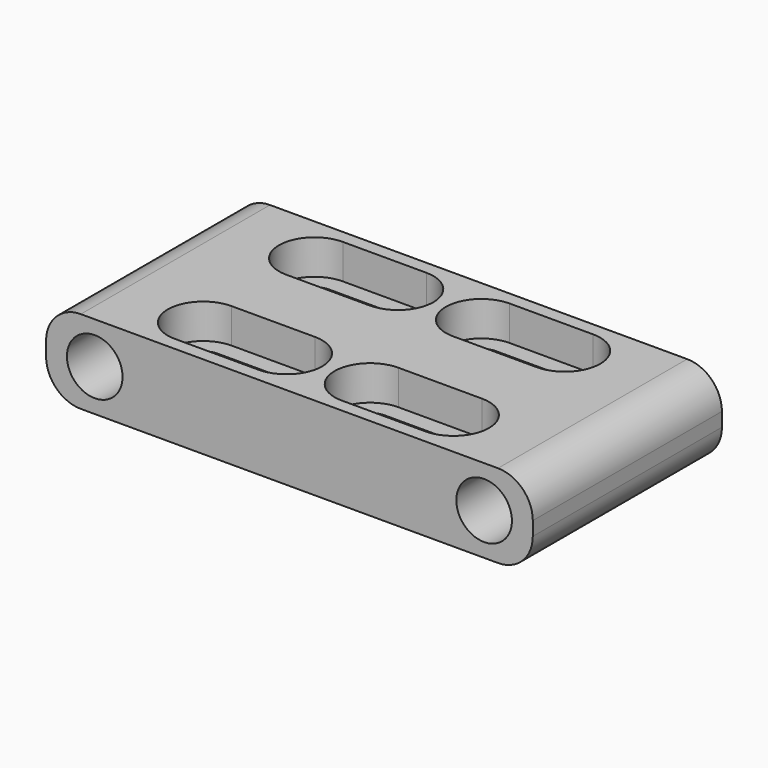
from build123d import *

# Parameters (mm, degrees)
F0_W     = 70
F0_H     = 34
F1_DEPTH = 12
F2_DEPTH = 7
F3_R     = 4
F4_DEPTH = 34.001
F5_R     = 5


# Not quite as in the source:
# - a feature names something its author has since deleted; it is built from what else it names


with BuildPart() as f1:
    # F0 (on Top) → F1 (new body)
    with BuildSketch(Plane.XY):
        Rectangle(F0_W, F0_H)
        with BuildLine():
            Line((-6, -15.1), (-18, -15.1))
            ThreePointArc((-18, -15.1), (-23.1, -10), (-18, -4.9))
            Line((-18, -4.9), (-6, -4.9))
            ThreePointArc((-6, -4.9), (-0.9, -10), (-6, -15.1))
        make_face(mode=Mode.SUBTRACT)
        with BuildLine():
            ThreePointArc((6, -15.1), (0.9, -10), (6, -4.9))
            Line((6, -4.9), (18, -4.9))
            ThreePointArc((18, -4.9), (23.1, -10), (18, -15.1))
            Line((18, -15.1), (6, -15.1))
        make_face(mode=Mode.SUBTRACT)
        with BuildLine():
            Line((-18, 15.1), (-6, 15.1))
            ThreePointArc((-6, 15.1), (-0.9, 10), (-6, 4.9))
            Line((-6, 4.9), (-18, 4.9))
            ThreePointArc((-18, 4.9), (-23.1, 10), (-18, 15.1))
        make_face(mode=Mode.SUBTRACT)
        with BuildLine():
            ThreePointArc((6, 4.9), (0.9, 10), (6, 15.1))
            Line((6, 15.1), (18, 15.1))
            ThreePointArc((18, 15.1), (23.1, 10), (18, 4.9))
            Line((18, 4.9), (6, 4.9))
        make_face(mode=Mode.SUBTRACT)
    extrude(amount=F1_DEPTH)

    # F0 (on Top) → F2 (join)
    with BuildSketch(Plane.XY):
        with BuildLine():
            ThreePointArc((-6, 4.9), (-0.9, 10), (-6, 15.1))
            Line((-6, 15.1), (-18, 15.1))
            ThreePointArc((-18, 15.1), (-23.1, 10), (-18, 4.9))
            Line((-18, 4.9), (-6, 4.9))
        make_face()
        with BuildLine():
            Line((-18, 12.6), (-6, 12.6))
            ThreePointArc((-6, 12.6), (-3.4, 10), (-6, 7.4))
            Line((-6, 7.4), (-18, 7.4))
            ThreePointArc((-18, 7.4), (-20.6, 10), (-18, 12.6))
        make_face(mode=Mode.SUBTRACT)
        with BuildLine():
            Line((18, 15.1), (6, 15.1))
            ThreePointArc((6, 15.1), (0.9, 10), (6, 4.9))
            Line((6, 4.9), (18, 4.9))
            ThreePointArc((18, 4.9), (23.1, 10), (18, 15.1))
        make_face()
        with BuildLine():
            ThreePointArc((6, 7.4), (3.4, 10), (6, 12.6))
            Line((6, 12.6), (18, 12.6))
            ThreePointArc((18, 12.6), (20.6, 10), (18, 7.4))
            Line((18, 7.4), (6, 7.4))
        make_face(mode=Mode.SUBTRACT)
        with BuildLine():
            Line((18, -4.9), (6, -4.9))
            ThreePointArc((6, -4.9), (0.9, -10), (6, -15.1))
            Line((6, -15.1), (18, -15.1))
            ThreePointArc((18, -15.1), (23.1, -10), (18, -4.9))
        make_face()
        with BuildLine():
            Line((18, -12.6), (6, -12.6))
            ThreePointArc((6, -12.6), (3.4, -10), (6, -7.4))
            Line((6, -7.4), (18, -7.4))
            ThreePointArc((18, -7.4), (20.6, -10), (18, -12.6))
        make_face(mode=Mode.SUBTRACT)
        with BuildLine():
            ThreePointArc((-18, -4.9), (-23.1, -10), (-18, -15.1))
            Line((-18, -15.1), (-6, -15.1))
            ThreePointArc((-6, -15.1), (-0.9, -10), (-6, -4.9))
            Line((-6, -4.9), (-18, -4.9))
        make_face()
        with BuildLine():
            Line((-6, -12.6), (-18, -12.6))
            ThreePointArc((-18, -12.6), (-20.6, -10), (-18, -7.4))
            Line((-18, -7.4), (-6, -7.4))
            ThreePointArc((-6, -7.4), (-3.4, -10), (-6, -12.6))
        make_face(mode=Mode.SUBTRACT)
    extrude(amount=F2_DEPTH)

    # F3 (on face) → F4 (cut, through all)
    with BuildSketch(Plane(origin=(0, 17, 0), x_dir=(-1, 0, 0), z_dir=(0, 1, 0))):
        with Locations((28, 6)):
            Circle(F3_R)
        with Locations((-28, 6)):
            Circle(F3_R)
    extrude(amount=-F4_DEPTH, mode=Mode.SUBTRACT)

    # F5
    f5_edges = [f1.edges().sort_by_distance(p)[0] for p in [
        (-35, 0, 12),
        (35, 0, 12),
        (-35, 0, 0),
        (35, 0, 0),
    ]]
    fillet(f5_edges, radius=F5_R)


solid = f1.part
